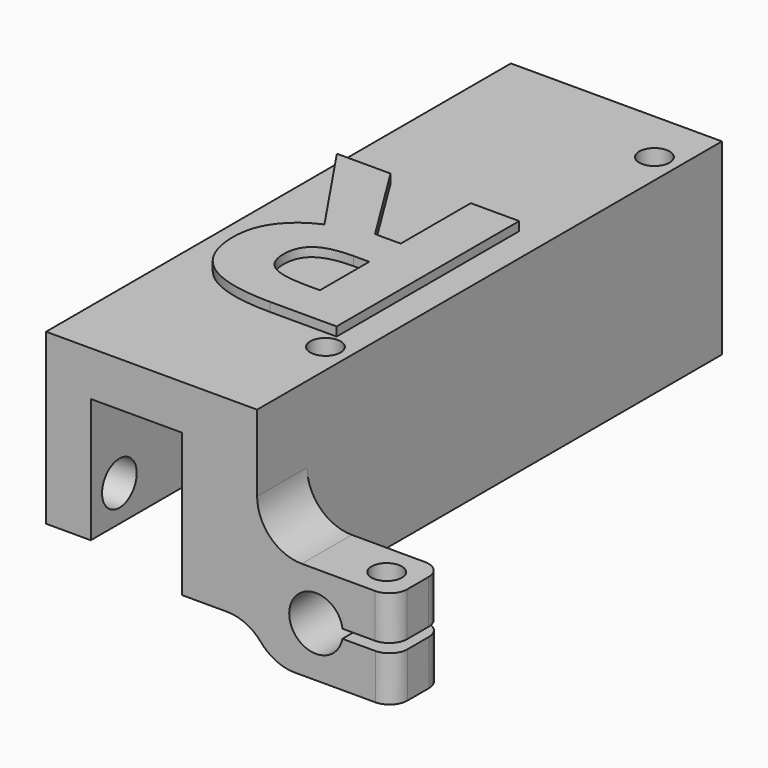
from build123d import *

# Parameters (mm, degrees)
F1_DEPTH      = 7
F2_DEPTH      = 58
F3_R          = 1.7
F3_R_2        = 11
F4_DEPTH      = 21.001
F5_R          = 3
F6_DEPTH      = 10
F7_DEPTH      = 21.001
F8_R          = 1.4
F9_DEPTH      = 11.0176173191
F8_R_2        = 1.7
F10_DEPTH     = 4.9119085967
F11_R         = 5
F12_R         = 5
F13_R         = 5
F14_R         = 2
F15_R         = 2.2
F15_R_2       = 2.4255023423
F16_DEPTH     = 6
F17_TEXT_SIZE = 35.7644961357
F18_DEPTH     = 1


# Not quite as in the source:
# - a feature names something its author has since deleted; it is built from what else it names
# - Text() gives the source's letters only with a copy of the font that has no kerning and outlines rounded to 1/6400 em; it was checked with that copy


with BuildPart() as f1:
    # F0 (on Front) → F1 (new body)
    with BuildSketch(Plane.XZ):
        Polygon((-18.6721007523, 29.8099789735), (-18.6721007523, 10.8925135386), (-13.6721007523, 10.8925135386), (-13.6721007523, 24.8099789735), (-3.4721007523, 24.8099789735), (-3.4721007523, 8.8099789735), (4.9380548998, 8.8099789735), (4.9380548998, 16.2656020473), (4.9380548998, 29.8099789735), align=None)
        Polygon((20.1263195603, 16.2417280634), (4.9380548998, 16.2656020473), (4.9380548998, 8.8099789735), (6.3533044869, 5.2860832236), (20.1553367778, 5.2860832236), (20.1553367778, 10.343908232), (13.4860510706, 10.343908232), (13.4860510706, 11.3388913612), (20.1263195603, 11.3388913612), align=None)
    extrude(amount=F1_DEPTH)

    # F0 (on Front) → F2 (join)
    with BuildSketch(Plane.XZ):
        Polygon((-18.6721007523, 29.8099789735), (-18.6721007523, 10.8925135386), (-13.6721007523, 10.8925135386), (-13.6721007523, 24.8099789735), (-3.4721007523, 24.8099789735), (-3.4721007523, 8.8099789735), (4.9380548998, 8.8099789735), (4.9380548998, 16.2656020473), (4.9380548998, 29.8099789735), align=None)
    extrude(amount=-F2_DEPTH)

    # F3 (on face) → F4 (cut, through all)
    with BuildSketch(Plane(origin=(0, 0, 8.8099789735), x_dir=(1, 0, 0), z_dir=(0, 0, -1))):
        with Locations((2.1850741468, -6)):
            Circle(F3_R)
        with Locations((2.1850741468, -52)):
            Circle(F3_R)
        with Locations((17.6850741468, -29)):
            Circle(F3_R_2)
    extrude(amount=-F4_DEPTH, mode=Mode.SUBTRACT)

    # F5 (on face) → F6 (cut)
    with BuildSketch(Plane.XZ.offset(7)):
        with Locations((11.5278992477, 10.8989789735)):
            Circle(F5_R)
    extrude(amount=-F6_DEPTH, mode=Mode.SUBTRACT)

    # F3 (on face) → F7 (cut, through all)
    with BuildSketch(Plane(origin=(0, 0, 8.8099789735), x_dir=(1, 0, 0), z_dir=(0, 0, -1))):
        with Locations((2.1850741468, -6)):
            Circle(F3_R)
        with Locations((2.1850741468, -52)):
            Circle(F3_R)
        with Locations((17.6850741468, -29)):
            Circle(F3_R_2)
    extrude(amount=-F7_DEPTH, mode=Mode.SUBTRACT)

    # F8 (on face) → F9 (cut, through all)
    with BuildSketch(Plane(origin=(0.0255795563, 0, 16.273323822), x_dir=(0.9999987646, 0, -0.0015718685), z_dir=(0.0015718685, 0, 0.9999987646))):
        with Locations((16.669401899, -3.5767070949)):
            Circle(F8_R)
    extrude(amount=-F9_DEPTH, mode=Mode.SUBTRACT)

    # F8 (on face) → F10 (cut, through all)
    with BuildSketch(Plane(origin=(0.0255795563, 0, 16.273323822), x_dir=(0.9999987646, 0, -0.0015718685), z_dir=(0.0015718685, 0, 0.9999987646))):
        with Locations((16.669401899, -3.5767070949)):
            Circle(F8_R_2)
        with Locations((16.669401899, -3.5767070949)):
            Circle(F8_R, mode=Mode.SUBTRACT)
    extrude(amount=-F10_DEPTH, mode=Mode.SUBTRACT)

    # F11
    f11_edges = [f1.edges().sort_by_distance(p)[0] for p in [
        (4.938055, -3.5, 16.265602),
    ]]
    fillet(f11_edges, radius=F11_R)

    # F12
    f12_edges = [f1.edges().sort_by_distance(p)[0] for p in [
        (4.938055, -3.5, 8.809979),
    ]]
    fillet(f12_edges, radius=F12_R)

    # F13
    f13_edges = [f1.edges().sort_by_distance(p)[0] for p in [
        (6.353304, -3.5, 5.286083),
    ]]
    fillet(f13_edges, radius=F13_R)

    # F14
    f14_edges = [f1.edges().sort_by_distance(p)[0] for p in [
        (20.12632, -7, 13.79031),
        (20.155337, -7, 7.814996),
        (20.12632, 0, 13.79031),
        (20.155337, 0, 7.814996),
    ]]
    fillet(f14_edges, radius=F14_R)

    # F15 (on face) → F16 (cut)
    with BuildSketch(Plane(origin=(-18.6721007523, 0, 0), x_dir=(0, -1, 0), z_dir=(-1, 0, 0))):
        with Locations((-54, 14.8925135386)):
            Circle(F15_R)
        with Locations((3, 14.8925135386)):
            Circle(F15_R_2)
    extrude(amount=-F16_DEPTH, mode=Mode.SUBTRACT)

    # F17 (on face) → F18 (join)
    with BuildSketch(Plane.XY.offset(29.8099789735)):
        with Locations(Location((4.9380548998, 33.6637421799), (0, 0, 180))):
            Text('R', F17_TEXT_SIZE, font='Open Sans', font_style=FontStyle.BOLD, text_align=(TextAlign.LEFT, TextAlign.BOTTOM))
    extrude(amount=F18_DEPTH)


solid = f1.part
